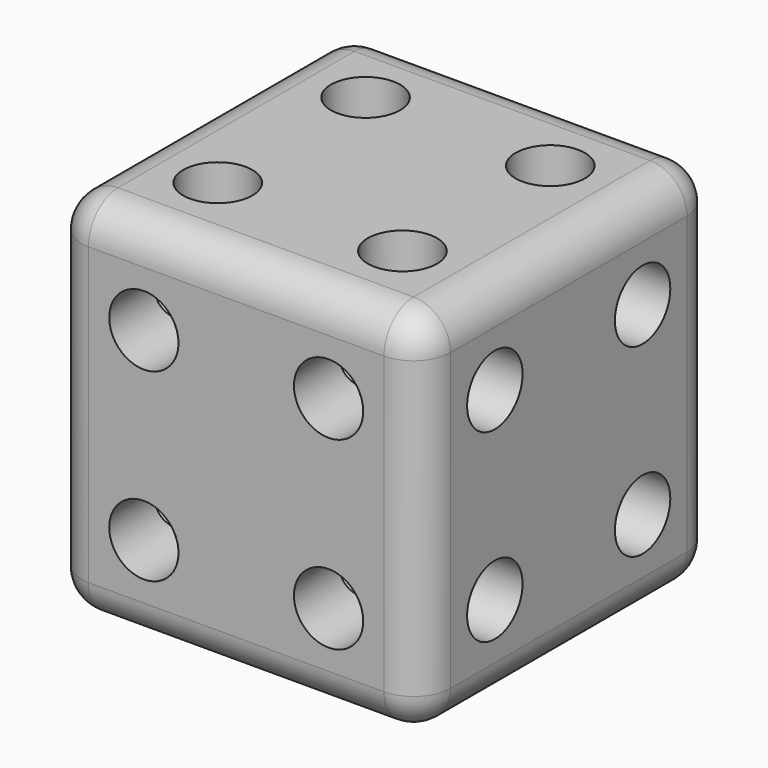
from build123d import *

# Parameters (mm, degrees)
F0_W     = 50.8
F0_H     = 50.8
F1_DEPTH = 50.8
F3_D     = 9.525
F4_D     = 9.525
F6_D     = 9.525
F7_R     = 5.08


# Not quite as in the source:
# - a length typed as a fraction of an inch, garbled in the dataset ("3 / 203.2 mm" for 3/8 in), is restored


with BuildPart() as f1:
    # F0 (on Front) → F1 (new body)
    with BuildSketch(Plane.XZ):
        with Locations((25.4, 25.4)):
            Rectangle(F0_W, F0_H)
    extrude(amount=F1_DEPTH)

    # F3 (through all)
    with Locations(Plane(origin=(0, 0, 0), x_dir=(0, -1, 0), z_dir=(-1, 0, 0))):
        with Locations((12.7, 38.1), (38.1, 38.1), (38.1, 12.7), (12.7, 12.7)):
            Hole(F3_D / 2)

    # F4 (through all)
    with Locations(Plane(origin=(0, 0, 0), x_dir=(1, 0, 0), z_dir=(0, 1, 0))):
        with Locations((38.1, -38.1), (12.7, -38.1), (12.7, -12.7), (38.1, -12.7)):
            Hole(F4_D / 2)

    # F6 (through all)
    with Locations(Plane.XY.offset(50.8)):
        with Locations((12.7, -12.7), (38.1, -12.7), (38.1, -38.1), (12.7, -38.1)):
            Hole(F6_D / 2)

    # F7
    f7_edges = [f1.edges().sort_by_distance(p)[0] for p in [
        (25.4, -50.8, 50.8),
        (0, -25.4, 50.8),
        (50.8, -25.4, 50.8),
        (25.4, 0, 50.8),
        (50.8, 0, 25.4),
        (0, 0, 25.4),
        (25.4, 0, 0),
        (50.8, -25.4, 0),
        (0, -25.4, 0),
        (25.4, -50.8, 0),
        (0, -50.8, 25.4),
        (50.8, -50.8, 25.4),
    ]]
    fillet(f7_edges, radius=F7_R)


solid = f1.part
